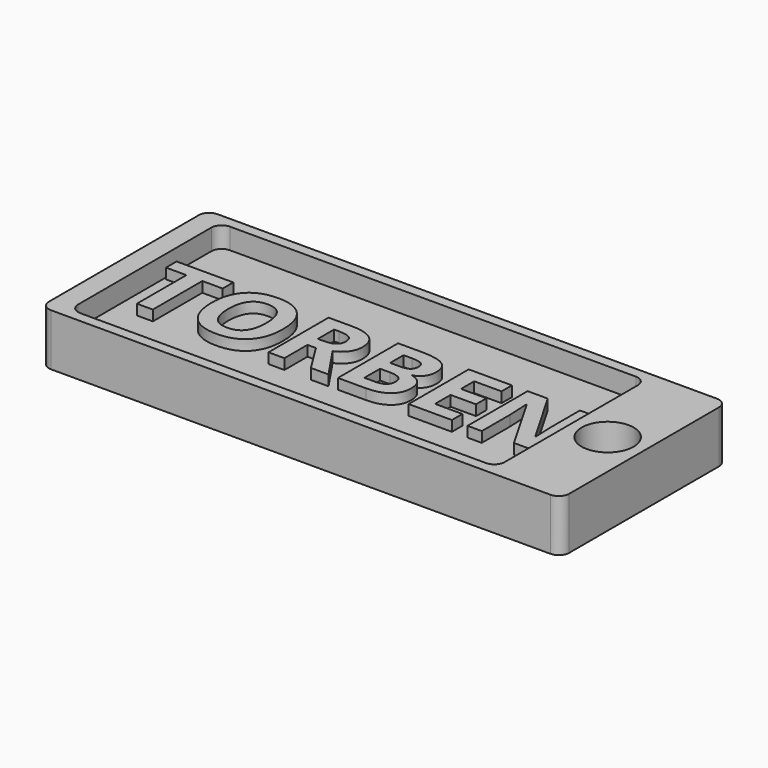
from build123d import *

# Parameters (mm, degrees)
F0_W         = 50
F0_H         = 20
F1_DEPTH     = 5
F2_W         = 41
F2_H         = 18
F3_DEPTH     = 2
F4_R         = 1
F5_R         = 1
F6_R         = 2.5
F7_DEPTH     = 25
F8_TEXT_SIZE = 10.110974106
F9_DEPTH     = 1


# Not quite as in the source:
# - Text() gives the source's letters only with a copy of the font that has no kerning and outlines rounded to 1/6400 em; it was checked with that copy


with BuildPart() as f1:
    # F0 (on Top) → F1 (new body)
    with BuildSketch(Plane.XY):
        with Locations((16.6330665722, -0.9630892425)):
            Rectangle(F0_W, F0_H)
    extrude(amount=F1_DEPTH)

    # F2 (on face) → F3 (cut)
    with BuildSketch(Plane.XY.offset(5)):
        with Locations((14.1330665722, -0.9630892425)):
            Rectangle(F2_W, F2_H)
    extrude(amount=-F3_DEPTH, mode=Mode.SUBTRACT)

    # F4
    f4_edges = [f1.edges().sort_by_distance(p)[0] for p in [
        (-8.366933, -10.963089, 2.5),
        (-8.366933, 9.036911, 2.5),
        (41.633067, -10.963089, 2.5),
        (41.633067, 9.036911, 2.5),
    ]]
    fillet(f4_edges, radius=F4_R)

    # F5
    f5_edges = [f1.edges().sort_by_distance(p)[0] for p in [
        (-6.366933, 8.036911, 4),
        (34.633067, 8.036911, 4),
        (-6.366933, -9.963089, 4),
        (34.633067, -9.963089, 4),
    ]]
    fillet(f5_edges, radius=F5_R)

    # F6 (on face) → F7 (cut)
    with BuildSketch(Plane.XY.offset(5)):
        with Locations((38.1330665722, -0.9630892425)):
            Circle(F6_R)
    extrude(amount=-F7_DEPTH, mode=Mode.SUBTRACT)

    # F8 (on face) → F9 (join)
    with BuildSketch(Plane.XY.offset(3)):
        with Locations((-6.3669334278, -4.6030399207)):
            Text('TORBEN', F8_TEXT_SIZE, font='Open Sans', font_style=FontStyle.BOLD, text_align=(TextAlign.LEFT, TextAlign.BOTTOM))
    extrude(amount=F9_DEPTH)


solid = f1.part
